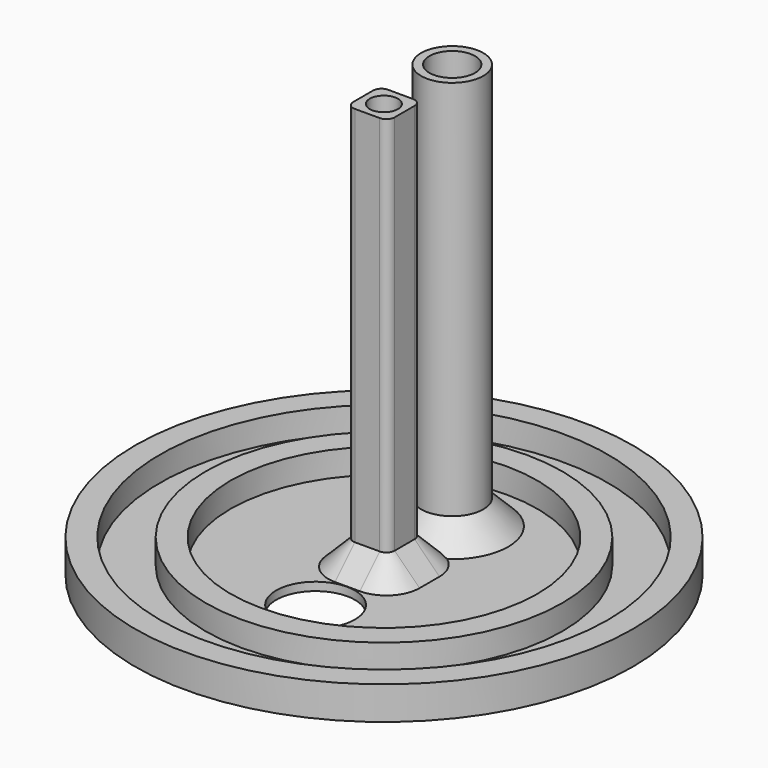
from build123d import *

# Parameters (mm, degrees)
F0_R         = 30
F0_R_2       = 27
F0_R_3       = 21.5
F0_R_4       = 18.5
F0_R_5       = 4.75
F0_W         = 5
F0_H         = 5
F0_R_6       = 3.75
F0_R_7       = 1.7
F1_DEPTH     = 1
F2_DEPTH     = 4
F0_R_8       = 2.75
F3_DEPTH     = 50
F4_R         = 1
F5_T1_DEPTH  = 3
F5_T3_DEPTH  = 3
F5_T6_ANGLE  = 90
F5_T10_ANGLE = 90
F5_T12_ANGLE = 90
F5_T14_ANGLE = 90


# Not quite as in the source:
# - a fillet or chamfer that OpenCascade refuses, or shapes differently, is made with other operations: its cross-section is extruded or revolved along the edge and cut away or added


with BuildPart() as f1:
    # F0 (on Top) → F1 (new body)
    with BuildSketch(Plane.XY):
        Circle(F0_R)
        Circle(F0_R_2, mode=Mode.SUBTRACT)
        Circle(F0_R_2)
        Circle(F0_R_3, mode=Mode.SUBTRACT)
        Circle(F0_R_3)
        Circle(F0_R_4, mode=Mode.SUBTRACT)
        Circle(F0_R_4)
        with Locations((0, -10.3181230716)):
            Circle(F0_R_5, mode=Mode.SUBTRACT)
        with Locations((0, -0.0181230716)):
            Rectangle(F0_W, F0_H, mode=Mode.SUBTRACT)
        with Locations((0, 10.2818769284)):
            Circle(F0_R_6, mode=Mode.SUBTRACT)
        with Locations((0, -0.0181230716)):
            Rectangle(F0_W, F0_H)
        with Locations((0, -0.0181230716)):
            Circle(F0_R_7, mode=Mode.SUBTRACT)
    extrude(amount=F1_DEPTH)

    # F0 (on Top) → F2 (join)
    with BuildSketch(Plane.XY):
        Circle(F0_R)
        Circle(F0_R_2, mode=Mode.SUBTRACT)
        Circle(F0_R_3)
        Circle(F0_R_4, mode=Mode.SUBTRACT)
    extrude(amount=F2_DEPTH)

    # F0 (on Top) → F3 (join)
    with BuildSketch(Plane.XY):
        with Locations((0, -0.0181230716)):
            Rectangle(F0_W, F0_H)
        with Locations((0, -0.0181230716)):
            Circle(F0_R_7, mode=Mode.SUBTRACT)
        with Locations((0, 10.2818769284)):
            Circle(F0_R_6)
        with Locations((0, 10.2818769284)):
            Circle(F0_R_8, mode=Mode.SUBTRACT)
    extrude(amount=F3_DEPTH)

    # F4
    f4_edges = [f1.edges().sort_by_distance(p)[0] for p in [
        (-2.5, -2.518123, 25.5),
        (2.5, -2.518123, 25.5),
        (-2.5, 2.481877, 25.5),
        (2.5, 2.481877, 25.5),
    ]]
    fillet(f4_edges, radius=F4_R)

    # F5: chamfer of 3 on 3 edges, made by hand

    # F5_s2 → F5_t1 (join)
    with BuildSketch(Plane.YZ.offset(-1.5)):
        Polygon((-5.5181230716, 1), (-2.5181230716, 4), (-2.5181230716, 1), align=None)
        Polygon((5.4818769284, 1), (2.4818769284, 4), (2.4818769284, 1), align=None)
    extrude(amount=F5_T1_DEPTH)

    # F5_s4 → F5_t3 (join)
    with BuildSketch(Plane.XZ.offset(-1.4818769284)):
        Polygon((-5.5, 1), (-2.5, 4), (-2.5, 1), align=None)
        Polygon((5.5, 1), (2.5, 4), (2.5, 1), align=None)
    extrude(amount=F5_T3_DEPTH)

    # F5_s5 → F5_t6 (revolve)
    with BuildSketch(Plane.YZ.offset(-1.5)):
        Polygon((-5.5181230716, 1), (-2.5181230716, 4), (-2.5181230716, 1), align=None)
    revolve(axis=Axis((-1.5, -1.5181230716, 1), (0, 0, -1)), revolution_arc=F5_T6_ANGLE)

    # F5_s7 → F5_t8 (revolve)
    with BuildSketch(Plane.XZ.offset(-10.2818769284)):
        Polygon((6.75, 1), (3.75, 4), (3.75, 1), align=None)
    revolve(axis=Axis((0, 10.2818769284, 1), (0, 0, 1)))

    # F5_s9 → F5_t10 (revolve)
    with BuildSketch(Plane.XZ.offset(-1.4818769284)):
        Polygon((-5.5, 1), (-2.5, 4), (-2.5, 1), align=None)
    revolve(axis=Axis((-1.5, 1.4818769284, 1), (0, 0, -1)), revolution_arc=F5_T10_ANGLE)

    # F5_s11 → F5_t12 (revolve)
    with BuildSketch(Plane.YZ.offset(1.5)):
        Polygon((5.4818769284, 1), (2.4818769284, 4), (2.4818769284, 1), align=None)
    revolve(axis=Axis((1.5, 1.4818769284, 1), (0, 0, -1)), revolution_arc=F5_T12_ANGLE)

    # F5_s13 → F5_t14 (revolve)
    with BuildSketch(Plane.YZ.offset(1.5)):
        Polygon((-5.5181230716, 1), (-2.5181230716, 4), (-2.5181230716, 1), align=None)
    revolve(axis=Axis((1.5, -1.5181230716, 1), (0, 0, 1)), revolution_arc=F5_T14_ANGLE)


solid = f1.part
